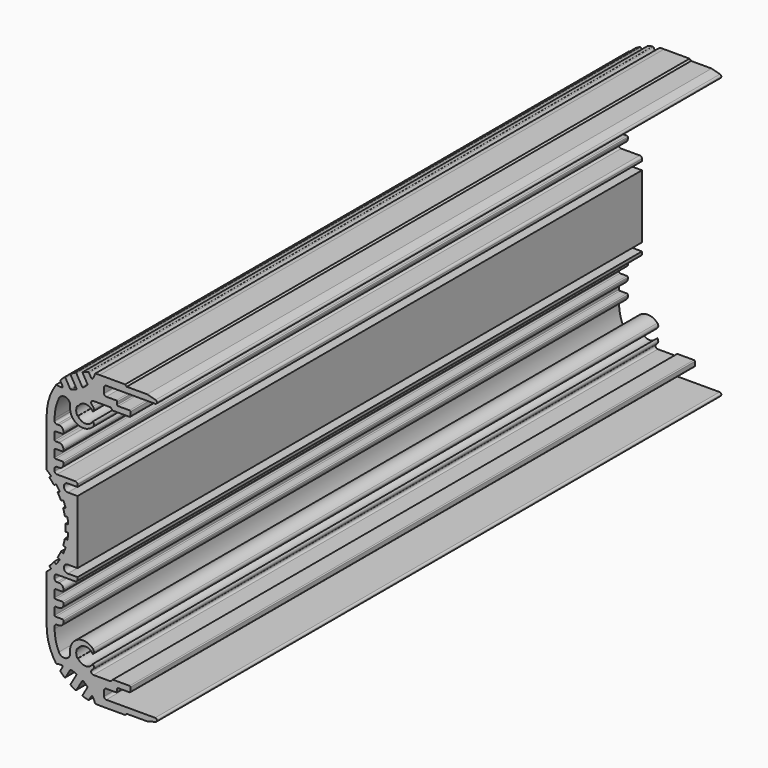
from build123d import *

# Parameters (mm, degrees)
F1_DEPTH = 160


# Not quite as in the source:
# - ends of sketch curves that miss each other by under 0.0002 mm in the source are joined


with BuildPart() as f1:
    # F0 (on Front) → F1 (new body)
    with BuildSketch(Plane.XZ):
        with BuildLine():
            ThreePointArc((-7.7, 7.2), (-8.6, 8.1), (-7.7, 9))
            Line((-7.7, 9), (-5.5, 9))
            Line((-5.5, 9), (-5.5, 9.5))
            ThreePointArc((-5.5, 9.5), (-5.6464466094, 9.8535533906), (-6, 10))
            Line((-6, 10), (-10.2, 10))
            ThreePointArc((-10.2, 10), (-10.5535533906, 10.1464466094), (-10.7, 10.5))
            Line((-10.7, 10.5), (-10.7, 11))
            ThreePointArc((-10.7, 11), (-10.5535533906, 11.3535533906), (-10.2, 11.5))
            Line((-10.2, 11.5), (-9.7, 11.5))
            ThreePointArc((-9.7, 11.5), (-8.9928932188, 11.7928932188), (-8.7, 12.5))
            Line((-8.7, 12.5), (-8.7, 12.8))
            ThreePointArc((-8.7, 12.8), (-8.7585786438, 12.9414213562), (-8.9, 13))
            Line((-8.9, 13), (-10.5, 13))
            ThreePointArc((-10.5, 13), (-10.6414213562, 13.0585786438), (-10.7, 13.2))
            Line((-10.7, 13.2), (-10.7, 14.8))
            ThreePointArc((-10.7, 14.8), (-10.6414213562, 14.9414213562), (-10.5, 15))
            Line((-10.5, 15), (-8.9, 15))
            ThreePointArc((-8.9, 15), (-8.7585786438, 15.0585786438), (-8.7, 15.2))
            Line((-8.7, 15.2), (-8.7, 15.5))
            ThreePointArc((-8.7, 15.5), (-8.9928932188, 16.2071067812), (-9.7, 16.5))
            Line((-9.7, 16.5), (-10.5, 16.5))
            ThreePointArc((-10.5, 16.5), (-10.6414213562, 16.5585786438), (-10.7, 16.7))
            Line((-10.7, 16.7), (-10.7, 18.3))
            ThreePointArc((-10.7, 18.3), (-10.6414213562, 18.4414213562), (-10.5, 18.5))
            Line((-10.5, 18.5), (-8.9, 18.5))
            ThreePointArc((-8.9, 18.5), (-8.7585786438, 18.5585786438), (-8.7, 18.7))
            Line((-8.7, 18.7), (-8.7, 19))
            ThreePointArc((-8.7, 19), (-8.9928932188, 19.7071067812), (-9.7, 20))
            Line((-9.7, 20), (-10.2, 20))
            ThreePointArc((-10.2, 20), (-10.5535533906, 20.1464466094), (-10.7, 20.5))
            Line((-10.7, 20.5), (-10.7, 21))
            ThreePointArc((-10.7, 21), (-10.4563998864, 23.2158748388), (-9.737235039, 25.3259090183))
            ThreePointArc((-9.737235039, 25.3259090183), (-8.1379919876, 26.0497497539), (-7.1756276034, 24.5816289491))
            ThreePointArc((-7.1756276034, 24.5816289491), (-5.4713643355, 21.4827159283), (-2.0002189991, 22.1601559991))
            ThreePointArc((-2.0002189991, 22.1601559991), (-1.8003504138, 22.686837824), (-2.0234984921, 23.2040865149))
            ThreePointArc((-2.0234984921, 23.2040865149), (-3.7121185112, 22.2500376563), (-5.388749653, 23.2250002003))
            Line((-5.388749653, 23.2250002003), (-5.518653, 23.15))
            ThreePointArc((-5.518653, 23.15), (-5.8, 24.2), (-5.518653261, 25.2500001507))
            Line((-5.518653261, 25.2500001507), (-5.38875, 25.175))
            ThreePointArc((-5.38875, 25.175), (-3.7121185112, 26.1499623437), (-2.0234990658, 25.1959139609))
            ThreePointArc((-2.0234990658, 25.1959139609), (-1.8003504138, 25.713162176), (-2.0002188653, 26.2398441249))
            ThreePointArc((-2.0002188653, 26.2398441249), (-2.1170146865, 26.3589747992), (-2.2402522096, 26.471428757))
            ThreePointArc((-2.2402522096, 26.471428757), (-2.3822876131, 27.0242332623), (-1.913627, 27.35))
            Line((-1.913627, 27.35), (2, 27.35))
            Line((2, 27.35), (2.5, 26.85))
            Line((2.5, 26.85), (6.3, 26.85))
            ThreePointArc((6.3, 26.85), (6.4414213562, 26.9085786438), (6.5, 27.05))
            Line((6.5, 27.05), (6.5, 27.95))
            ThreePointArc((6.5, 27.95), (6.4414213562, 28.0914213562), (6.3, 28.15))
            Line((6.3, 28.15), (3.7, 28.15))
            ThreePointArc((3.7, 28.15), (3.5585786438, 28.2085786438), (3.5, 28.35))
            Line((3.5, 28.35), (3.5, 28.95))
            ThreePointArc((3.5, 28.95), (3.4414213562, 29.0914213562), (3.3, 29.15))
            Line((3.3, 29.15), (1, 29.15))
            ThreePointArc((1, 29.15), (0.6464466094, 29.2964466094), (0.5, 29.65))
            Line((0.5, 29.65), (0.5, 30.85))
            ThreePointArc((0.5, 30.85), (0.6464466094, 31.2035533906), (1, 31.35))
            Line((1, 31.35), (12.1, 31.35))
            ThreePointArc((12.1, 31.35), (12.4965779149, 31.6977892978), (12.203528057, 32.1363702129))
            Line((12.203528057, 32.1363702129), (10.286636, 32.65))
            Line((10.286636, 32.65), (5.65, 32.65))
            Line((5.65, 32.65), (5.3, 33))
            Line((5.3, 33), (-0.5, 33))
            ThreePointArc((-0.5, 33), (-0.9962043804, 32.9897364947), (-1.4915599615, 32.9589635355))
            ThreePointArc((-1.4915599615, 32.9589635355), (-1.7420019294, 32.3552616733), (-2.0408889921, 31.7740179955))
            ThreePointArc((-2.0408889921, 31.7740179955), (-2.2140891786, 31.6726695125), (-2.3880720606, 31.772667965))
            Line((-2.3880720606, 31.772667965), (-2.877826, 32.620948))
            ThreePointArc((-2.877826, 32.620948), (-2.9704583056, 32.704000017), (-3.0942690554, 32.7162182501))
            ThreePointArc((-3.0942690554, 32.7162182501), (-3.6559634907, 32.5775599521), (-4.2103219342, 32.4119897978))
            ThreePointArc((-4.2103219342, 32.4119897978), (-4.3352057845, 32.2934461354), (-4.3216880606, 32.121789965))
            Line((-4.3216880606, 32.121789965), (-3.286774, 30.329266))
            ThreePointArc((-3.286774, 30.329266), (-3.2616322345, 30.2036035638), (-3.3179275562, 30.0884775512))
            ThreePointArc((-3.3179275562, 30.0884775512), (-3.7373321665, 29.6946927651), (-4.183952239, 29.3320673169))
            ThreePointArc((-4.183952239, 29.3320673169), (-4.3442040216, 29.2957762661), (-4.4775590606, 29.391765965))
            Line((-4.4775590606, 29.391765965), (-5.742987, 31.583552))
            ThreePointArc((-5.742987, 31.583552), (-5.8599290844, 31.6754751209), (-6.0079921033, 31.6612392))
            ThreePointArc((-6.0079921033, 31.6612392), (-6.4999999515, 31.3923048734), (-6.9789078755, 31.1006808058))
            ThreePointArc((-6.9789078755, 31.1006808058), (-7.0652677962, 30.9795722811), (-7.0441310606, 30.832335965))
            Line((-7.0441310606, 30.832335965), (-5.778553, 28.640291))
            ThreePointArc((-5.778553, 28.640291), (-5.762090881, 28.4768372061), (-5.8735979557, 28.3561958956))
            ThreePointArc((-5.8735979557, 28.3561958956), (-6.4108526699, 28.1505669893), (-6.9614951162, 27.984077441))
            ThreePointArc((-6.9614951162, 27.984077441), (-7.0893773889, 27.9928590787), (-7.1856630606, 28.077475965))
            Line((-7.1856630606, 28.077475965), (-8.220909, 29.870574))
            ThreePointArc((-8.220909, 29.870574), (-8.3628085339, 29.9681087255), (-8.5279121396, 29.9192281551))
            ThreePointArc((-8.5279121396, 29.9192281551), (-8.9484792284, 29.5219245906), (-9.3494080152, 29.1048120139))
            ThreePointArc((-9.3494080152, 29.1048120139), (-9.4007320648, 28.9914798188), (-9.3751230606, 28.869731965))
            Line((-9.3751230606, 28.869731965), (-8.884654, 28.020215))
            ThreePointArc((-8.884654, 28.020215), (-8.8850258511, 27.8195735441), (-9.0593419963, 27.7202204983))
            ThreePointArc((-9.0593419963, 27.7202204983), (-9.7130395317, 27.7518399473), (-10.361965044, 27.8367867453))
            ThreePointArc((-10.361965044, 27.8367867453), (-11.9530252735, 24.5816493525), (-12.5, 21))
            Line((-12.5, 21), (-12.5, 10.132527))
            ThreePointArc((-12.5, 10.132527), (-11.9817250184, 9.7008809568), (-11.486700928, 9.2427560738))
            Line((-11.486700928, 9.2427560738), (-11.891636, 8.827512))
            ThreePointArc((-11.891636, 8.827512), (-11.3370242501, 8.2503803189), (-10.8210268423, 7.6384801245))
            Line((-10.8210268423, 7.6384801245), (-10.365731, 7.997792))
            ThreePointArc((-10.365731, 7.997792), (-9.9247470382, 7.4048716933), (-9.5184091179, 6.7876919271))
            Line((-9.5184091179, 6.7876919271), (-10.011773, 6.482745))
            ThreePointArc((-10.011773, 6.482745), (-9.613256057, 5.7885841377), (-9.2606180666, 5.0700289699))
            Line((-9.2606180666, 5.0700289699), (-8.731921, 5.308522))
            ThreePointArc((-8.731921, 5.308522), (-8.4474766389, 4.6265300852), (-8.2025179477, 3.9293810167))
            Line((-8.2025179477, 3.9293810167), (-8.755, 3.752848))
            ThreePointArc((-8.755, 3.752848), (-8.5362536455, 2.982896774), (-8.3679247585, 2.2003750438))
            Line((-8.3679247585, 2.2003750438), (-7.797235, 2.30388))
            ThreePointArc((-7.797235, 2.30388), (-7.6862291765, 1.5733331759), (-7.6172024513, 0.8376319707))
            Line((-7.6172024513, 0.8376319707), (-8.19598, 0.8))
            ThreePointArc((-8.19598, 0.8), (-8.17, 0), (-8.1959803302, -0.7999999785))
            Line((-8.1959803302, -0.7999999785), (-7.617202, -0.837632))
            ThreePointArc((-7.617202, -0.837632), (-7.6862291765, -1.5733331759), (-7.7972350648, -2.3038799883))
            Line((-7.7972350648, -2.3038799883), (-8.367925, -2.200375))
            ThreePointArc((-8.367925, -2.200375), (-8.5362536455, -2.982896774), (-8.7549997339, -3.752848085))
            Line((-8.7549997339, -3.752848085), (-8.202518, -3.929381))
            ThreePointArc((-8.202518, -3.929381), (-8.4474766389, -4.6265300852), (-8.7319206178, -5.3085221724))
            Line((-8.7319206178, -5.3085221724), (-9.260618, -5.070029))
            ThreePointArc((-9.260618, -5.070029), (-9.613256057, -5.7885841377), (-10.0117725977, -6.4827452486))
            Line((-10.0117725977, -6.4827452486), (-9.518409, -6.787692))
            ThreePointArc((-9.518409, -6.787692), (-9.9247470382, -7.4048716933), (-10.3657305452, -7.9977923589))
            Line((-10.3657305452, -7.9977923589), (-10.821027, -7.63848))
            ThreePointArc((-10.821027, -7.63848), (-11.3370242501, -8.2503803189), (-11.8916359679, -8.8275120329))
            Line((-11.8916359679, -8.8275120329), (-11.486701, -9.242756))
            ThreePointArc((-11.486701, -9.242756), (-11.9817250184, -9.7008809568), (-12.5000000817, -10.1325268965))
            Line((-12.5000000817, -10.1325268965), (-12.5, -21))
            ThreePointArc((-12.5, -21), (-11.9530252735, -24.5816493525), (-10.3619646526, -27.8367867592))
            ThreePointArc((-10.3619646526, -27.8367867592), (-9.7130395317, -27.7518399473), (-9.0593419993, -27.7202200951))
            ThreePointArc((-9.0593419993, -27.7202200951), (-8.8850258511, -27.8195735441), (-8.8846539394, -28.020215035))
            Line((-8.8846539394, -28.020215035), (-9.375123, -28.869732))
            ThreePointArc((-9.375123, -28.869732), (-9.4007320648, -28.9914798188), (-9.3494081724, -29.1048121579))
            ThreePointArc((-9.3494081724, -29.1048121579), (-8.9484792284, -29.5219245906), (-8.5279120224, -29.9192280249))
            ThreePointArc((-8.5279120224, -29.9192280249), (-8.3628085339, -29.9681087255), (-8.2209089394, -29.870574035))
            Line((-8.2209089394, -29.870574035), (-7.185663, -28.077476))
            ThreePointArc((-7.185663, -28.077476), (-7.0893773889, -27.9928590787), (-6.9614952552, -27.9840779684))
            ThreePointArc((-6.9614952552, -27.9840779684), (-6.4108526699, -28.1505669893), (-5.8735979711, -28.3561959319))
            ThreePointArc((-5.8735979711, -28.3561959319), (-5.762090881, -28.4768372061), (-5.7785529394, -28.640291035))
            Line((-5.7785529394, -28.640291035), (-7.044131, -30.832336))
            ThreePointArc((-7.044131, -30.832336), (-7.0652677962, -30.9795722811), (-6.9789077957, -31.1006806815))
            ThreePointArc((-6.9789077957, -31.1006806815), (-6.4999999515, -31.3923048734), (-6.007992136, -31.6612392633))
            ThreePointArc((-6.007992136, -31.6612392633), (-5.8599290844, -31.6754751209), (-5.7429869394, -31.583552035))
            Line((-5.7429869394, -31.583552035), (-4.477559, -29.391766))
            ThreePointArc((-4.477559, -29.391766), (-4.3442040216, -29.2957762661), (-4.1839526204, -29.3320678229))
            ThreePointArc((-4.1839526204, -29.3320678229), (-3.7373321665, -29.6946927651), (-3.3179272165, -30.0884772146))
            ThreePointArc((-3.3179272165, -30.0884772146), (-3.2616322345, -30.2036035638), (-3.2867739394, -30.329266035))
            Line((-3.2867739394, -30.329266035), (-4.321688, -32.12179))
            ThreePointArc((-4.321688, -32.12179), (-4.3352057845, -32.2934461354), (-4.2103219212, -32.4119897577))
            ThreePointArc((-4.2103219212, -32.4119897577), (-3.6559634907, -32.5775599521), (-3.0942690372, -32.7162181681))
            ThreePointArc((-3.0942690372, -32.7162181681), (-2.9704583056, -32.704000017), (-2.8778259394, -32.620948035))
            Line((-2.8778259394, -32.620948035), (-2.388072, -31.772668))
            ThreePointArc((-2.388072, -31.772668), (-2.2140891786, -31.6726695125), (-2.0408893631, -31.7740182059))
            ThreePointArc((-2.0408893631, -31.7740182059), (-1.7420019294, -32.3552616733), (-1.4915594736, -32.9589638064))
            ThreePointArc((-1.4915594736, -32.9589638064), (-0.9962043804, -32.9897364947), (-0.5, -33))
            Line((-0.5, -33), (5.3, -33))
            Line((5.3, -33), (5.65, -32.65))
            Line((5.65, -32.65), (10.286636, -32.65))
            Line((10.286636, -32.65), (12.203528, -32.13637))
            ThreePointArc((12.203528, -32.13637), (12.4965779149, -31.6977892978), (12.1, -31.35))
            Line((12.1, -31.35), (1, -31.35))
            ThreePointArc((1, -31.35), (0.6464466094, -31.2035533906), (0.5, -30.85))
            Line((0.5, -30.85), (0.5, -29.65))
            ThreePointArc((0.5, -29.65), (0.6464466094, -29.2964466094), (1, -29.15))
            Line((1, -29.15), (3.3, -29.15))
            ThreePointArc((3.3, -29.15), (3.4414213562, -29.0914213562), (3.5, -28.95))
            Line((3.5, -28.95), (3.5, -28.35))
            ThreePointArc((3.5, -28.35), (3.5585786438, -28.2085786438), (3.7, -28.15))
            Line((3.7, -28.15), (6.3, -28.15))
            ThreePointArc((6.3, -28.15), (6.4414213562, -28.0914213562), (6.5, -27.95))
            Line((6.5, -27.95), (6.5, -27.05))
            ThreePointArc((6.5, -27.05), (6.4414213562, -26.9085786438), (6.3, -26.85))
            Line((6.3, -26.85), (2.5, -26.85))
            Line((2.5, -26.85), (2, -27.35))
            Line((2, -27.35), (-1.913627, -27.35))
            ThreePointArc((-1.913627, -27.35), (-2.3822876131, -27.0242332623), (-2.2402520701, -26.4714289187))
            ThreePointArc((-2.2402520701, -26.4714289187), (-2.1170146865, -26.3589747992), (-2.0002189991, -26.2398440009))
            ThreePointArc((-2.0002189991, -26.2398440009), (-1.8003504138, -25.713162176), (-2.0234984921, -25.1959134851))
            ThreePointArc((-2.0234984921, -25.1959134851), (-3.7121185112, -26.1499623437), (-5.388749653, -25.1749997997))
            Line((-5.388749653, -25.1749997997), (-5.518653, -25.25))
            ThreePointArc((-5.518653, -25.25), (-5.8, -24.2), (-5.518653261, -23.1499998493))
            Line((-5.518653261, -23.1499998493), (-5.38875, -23.225))
            ThreePointArc((-5.38875, -23.225), (-3.7121185112, -22.2500376563), (-2.0234990658, -23.2040860391))
            ThreePointArc((-2.0234990658, -23.2040860391), (-1.8003504138, -22.686837824), (-2.0002188653, -22.1601558751))
            ThreePointArc((-2.0002188653, -22.1601558751), (-5.4713643355, -21.4827159283), (-7.1756275556, -24.581628943))
            ThreePointArc((-7.1756275556, -24.581628943), (-8.1379919876, -26.0497497539), (-9.7372351013, -25.3259090475))
            ThreePointArc((-9.7372351013, -25.3259090475), (-10.4563998864, -23.2158748388), (-10.7, -21))
            Line((-10.7, -21), (-10.7, -20.5))
            ThreePointArc((-10.7, -20.5), (-10.5535533906, -20.1464466094), (-10.2, -20))
            Line((-10.2, -20), (-9.7, -20))
            ThreePointArc((-9.7, -20), (-8.9928932188, -19.7071067812), (-8.7, -19))
            Line((-8.7, -19), (-8.7, -18.7))
            ThreePointArc((-8.7, -18.7), (-8.7585786438, -18.5585786438), (-8.9, -18.5))
            Line((-8.9, -18.5), (-10.5, -18.5))
            ThreePointArc((-10.5, -18.5), (-10.6414213562, -18.4414213562), (-10.7, -18.3))
            Line((-10.7, -18.3), (-10.7, -16.7))
            ThreePointArc((-10.7, -16.7), (-10.6414213562, -16.5585786438), (-10.5, -16.5))
            Line((-10.5, -16.5), (-9.7, -16.5))
            ThreePointArc((-9.7, -16.5), (-8.9928932188, -16.2071067812), (-8.7, -15.5))
            Line((-8.7, -15.5), (-8.7, -15.2))
            ThreePointArc((-8.7, -15.2), (-8.7585786438, -15.0585786438), (-8.9, -15))
            Line((-8.9, -15), (-10.5, -15))
            ThreePointArc((-10.5, -15), (-10.6414213562, -14.9414213562), (-10.7, -14.8))
            Line((-10.7, -14.8), (-10.7, -13.2))
            ThreePointArc((-10.7, -13.2), (-10.6414213562, -13.0585786438), (-10.5, -13))
            Line((-10.5, -13), (-8.9, -13))
            ThreePointArc((-8.9, -13), (-8.7585786438, -12.9414213562), (-8.7, -12.8))
            Line((-8.7, -12.8), (-8.7, -12.5))
            ThreePointArc((-8.7, -12.5), (-8.9928932188, -11.7928932188), (-9.7, -11.5))
            Line((-9.7, -11.5), (-10.2, -11.5))
            ThreePointArc((-10.2, -11.5), (-10.5535533906, -11.3535533906), (-10.7, -11))
            Line((-10.7, -11), (-10.7, -10.5))
            ThreePointArc((-10.7, -10.5), (-10.5535533906, -10.1464466094), (-10.2, -10))
            Line((-10.2, -10), (-6, -10))
            ThreePointArc((-6, -10), (-5.6464466094, -9.8535533906), (-5.5, -9.5))
            Line((-5.5, -9.5), (-5.5, -9))
            Line((-5.5, -9), (-7.7, -9))
            ThreePointArc((-7.7, -9), (-8.6, -8.1), (-7.7, -7.2))
            Line((-7.7, -7.2), (-5.5, -7.2))
            Line((-5.5, -7.2), (-5.5, 7.2))
            Line((-5.5, 7.2), (-7.7, 7.2))
        make_face()
    extrude(amount=F1_DEPTH)


solid = f1.part
